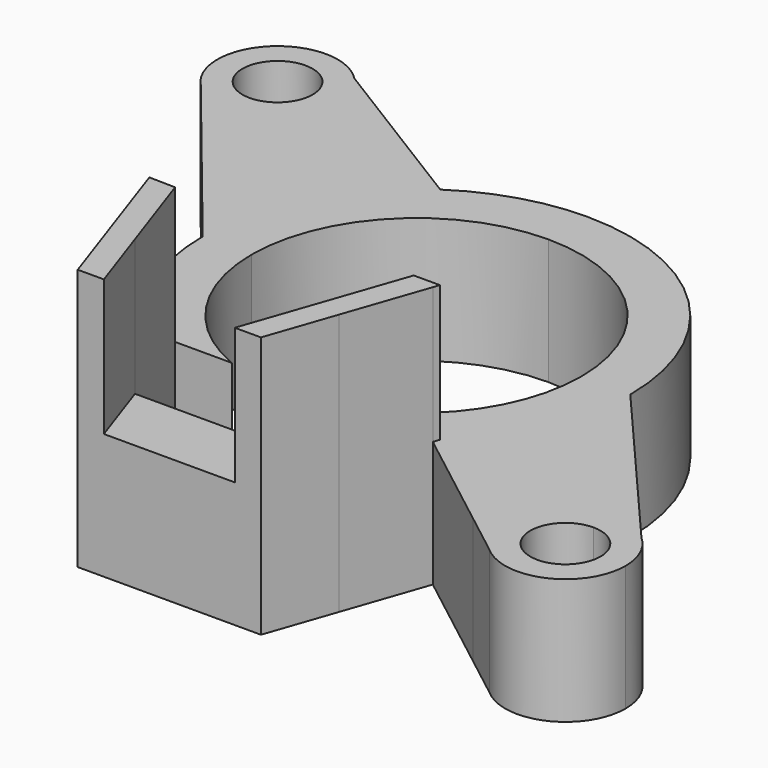
from build123d import *

# Parameters (mm, degrees)
F1_DEPTH = 12
F2_DEPTH = 25
F3_DEPTH = 12


# Not quite as in the source:
# - ends of sketch curves that miss each other by under 0.0002 mm in the source are joined


with BuildPart() as f1:
    # F0 (on Top) → F1 (new body)
    with BuildSketch(Plane.XY):
        with BuildLine():
            ThreePointArc((-53.4150354708, 40.5196217052), (-52.7133447942, 39.4447339634), (-52.4674114416, 38.1848648238))
            Line((-52.4674114416, 38.1848648238), (-50.0674114416, 38.1848649627))
            ThreePointArc((-50.0674114416, 38.1848649627), (-50.4895358529, 40.3473267799), (-51.6939302977, 42.1922833515))
            Line((-51.6939302977, 42.1922833515), (-53.4150354708, 40.5196217052))
        make_face()
        with BuildLine():
            Line((-50.0674114416, 38.1848649627), (-52.4674114416, 38.1848649047))
            ThreePointArc((-52.4674114416, 38.1848649047), (-53.4486037246, 35.8160571069), (-55.8174114415, 34.8348648238))
            Line((-55.8174114415, 34.8348648238), (-55.8174114415, 32.4348648238))
            ThreePointArc((-55.8174114415, 32.4348648238), (-51.7515474497, 34.119000832), (-50.0674114416, 38.1848649627))
        make_face()
        with BuildLine():
            ThreePointArc((-51.6939302977, 42.1922833515), (-50.4895358529, 40.3473267799), (-50.0674114416, 38.1848648238))
            Line((-50.0674114416, 38.1848648238), (-45.2079510631, 38.1848650801))
            Line((-45.2079510631, 38.1848650801), (-51.6939302977, 42.1922833515))
        make_face()
        with BuildLine():
            Line((-45.2079510631, 38.1848650801), (-50.0674114416, 38.1848649627))
            ThreePointArc((-50.0674114416, 38.1848649627), (-51.7515474497, 34.119000832), (-55.8174114415, 32.4348648238))
            Line((-55.8174114415, 32.4348648238), (-55.8174114414, 29.083605512))
            Line((-55.8174114414, 29.083605512), (-44.5532578407, 15.1687110318))
            ThreePointArc((-44.5532578407, 15.1687110318), (-42.1350647352, 24.8048651036), (-35.4555304308, 32.1592477879))
            Line((-35.4555304308, 32.1592477879), (-45.2079510631, 38.1848650801))
        make_face()
        with BuildLine():
            Line((-55.8174114415, 32.4348648238), (-55.8174114415, 34.8348648238))
            ThreePointArc((-55.8174114415, 34.8348648238), (-57.1214560051, 35.0990962362), (-58.2197874124, 35.8501079425))
            Line((-58.2197874124, 35.8501079425), (-59.9408925855, 34.1774462962))
            ThreePointArc((-59.9408925855, 34.1774462962), (-58.0556968865, 32.8883963526), (-55.8174114415, 32.4348648238))
        make_face()
        with BuildLine():
            ThreePointArc((-58.2197874124, 35.8501079425), (-58.1521683229, 40.5872407946), (-53.4150354708, 40.5196217052))
            Line((-53.4150354708, 40.5196217052), (-51.6939302977, 42.1922833515))
            ThreePointArc((-51.6939302977, 42.1922833515), (-59.8248299692, 42.3083459677), (-59.9408925855, 34.1774462962))
            Line((-59.9408925855, 34.1774462962), (-58.2197874124, 35.8501079425))
        make_face()
        with BuildLine():
            Line((-55.8174114414, 29.083605512), (-55.8174114415, 32.4348648238))
            ThreePointArc((-55.8174114415, 32.4348648238), (-58.0556968865, 32.8883963526), (-59.9408925855, 34.1774462962))
            Line((-59.9408925855, 34.1774462962), (-55.8174114414, 29.083605512))
        make_face()
        with BuildLine():
            ThreePointArc((-24.1338443596, 35.5853722206), (-30.0482104313, 34.7100811604), (-35.4555304308, 32.1592477879))
            ThreePointArc((-35.4555304308, 32.1592477879), (-42.1350647352, 24.8048651036), (-44.5532578407, 15.1687110318))
            Line((-44.5532578407, 15.1687110318), (-42.6338443592, 15.1659585535))
            Line((-42.6338443592, 15.1659585535), (-39.8838443592, 15.1659585535))
            ThreePointArc((-39.8838443592, 15.1659585535), (-35.270776163, 26.3028903571), (-24.1338443595, 30.9159585535))
            Line((-24.1338443595, 30.9159585535), (-24.1338443596, 35.5853722206))
        make_face()
        with BuildLine():
            ThreePointArc((-3.7144306922, 15.1659585535), (-9.6951384875, 29.6046644255), (-24.1338443596, 35.5853722206))
            Line((-24.1338443596, 35.5853722206), (-24.1338443595, 30.9159585535))
            ThreePointArc((-24.1338443595, 30.9159585535), (-12.9969125556, 26.3028903573), (-8.3838443592, 15.1659585535))
            Line((-8.3838443592, 15.1659585535), (-5.6338443592, 15.1659585535))
            Line((-5.6338443592, 15.1659585535), (-3.7144306922, 15.1659585535))
        make_face()
        with BuildLine():
            Line((-42.6338443592, 15.1659585535), (-44.5532578407, 15.1687110318))
            ThreePointArc((-44.5532578407, 15.1687110318), (-42.7914410163, 6.8685769492), (-37.807970261, 0.0011725238))
            Line((-37.807970261, 0.0011725238), (-38.0284454354, 0.643162408))
            Line((-38.0284454354, 0.643162408), (-35.5289696075, 0.5919707473))
            Line((-35.5289696075, 0.5919707473), (-42.6338443592, 15.1659585535))
        make_face()
        with BuildLine():
            Line((7.5497227229, 2.079326472), (-3.7144306922, 15.1659585535))
            Line((-3.7144306922, 15.1659585535), (-5.6338443592, 15.1659585535))
            Line((-5.6338443592, 15.1659585535), (-12.7387191109, 0.5919707473))
            Line((-12.7387191109, 0.5919707473), (-10.2387191109, 0.5919707473))
            Line((-10.2387191109, 0.5919707473), (-10.4427343672, 0))
            Line((-10.4427343672, 0), (-0.3331204375, -7.8151351762))
            Line((-0.3331204375, -7.8151351762), (1.9170354556, -7.8151351762))
            ThreePointArc((1.9170354556, -7.8151351762), (3.0939956275, -3.0251503303), (7.549722723, -0.909568585))
            Line((7.549722723, -0.909568585), (7.5497227229, 2.079326472))
        make_face()
        with BuildLine():
            Line((-39.8838443592, 15.1659585535), (-42.6338443592, 15.1659585535))
            Line((-42.6338443592, 15.1659585535), (-35.5289696075, 0.5919707473))
            Line((-35.5289696075, 0.5919707473), (-30.1055593076, 0.5919707473))
            ThreePointArc((-30.1055593076, 0.5919707473), (-37.2127780015, 6.3907665453), (-39.8838443592, 15.1659585535))
        make_face()
        Polygon((-38.0284454354, 0.643162408), (-37.807970261, 0.0011725238), (-35.1236572441, -7.8151351762), (-32.6315665225, -7.8151351762), (-35.5289696075, 0.5919707473), align=None)
        with BuildLine():
            Line((-5.6338443592, 15.1659585535), (-8.3838443592, 15.1659585535))
            ThreePointArc((-8.3838443592, 15.1659585535), (-11.054910717, 6.3907665453), (-18.1621294109, 0.5919707473))
            Line((-18.1621294109, 0.5919707473), (-12.7387191109, 0.5919707473))
            Line((-12.7387191109, 0.5919707473), (-5.6338443592, 15.1659585535))
        make_face()
        with BuildLine():
            Line((11.3813838275, -2.3722765282), (7.5497227229, 2.079326472))
            Line((7.5497227229, 2.079326472), (7.549722723, -0.909568585))
            ThreePointArc((7.549722723, -0.909568585), (9.6004019609, -1.2876774223), (11.3813838275, -2.3722765282))
        make_face()
        Polygon((-32.6315665225, -7.8151351762), (-35.1236572441, -7.8151351762), (-32.8838443592, -14.3371266833), (-30.3838443592, -14.3371266833), align=None)
        Polygon((-10.2387191109, 0.5919707473), (-12.7387191109, 0.5919707473), (-15.636122196, -7.8151351762), (-13.136122196, -7.8151351762), (-10.4427343672, 0), align=None)
        with BuildLine():
            ThreePointArc((11.3813838275, -2.3722765282), (9.6004019609, -1.2876774223), (7.549722723, -0.909568585))
            Line((7.549722723, -0.909568585), (7.549722723, -3.309568585))
            ThreePointArc((7.549722723, -3.309568585), (8.744466279, -3.5298580815), (9.7820818013, -4.1617549519))
            Line((9.7820818013, -4.1617549519), (11.3813838275, -2.3722765282))
        make_face()
        with BuildLine():
            Line((7.549722723, -3.309568585), (7.549722723, -0.909568585))
            ThreePointArc((7.549722723, -0.909568585), (3.0939956275, -3.0251503303), (1.9170354556, -7.8151351762))
            ThreePointArc((1.9170354556, -7.8151351762), (2.5652068364, -9.5261172721), (3.7180616186, -10.9468606418))
            Line((3.7180616186, -10.9468606418), (5.3173636448, -9.1573822181))
            ThreePointArc((5.3173636448, -9.1573822181), (4.4200122196, -5.464825029), (7.549722723, -3.309568585))
        make_face()
        with BuildLine():
            ThreePointArc((13.2997227231, -6.659568585), (12.7982725871, -4.3111171112), (11.3813838275, -2.3722765282))
            Line((11.3813838275, -2.3722765282), (9.7820818013, -4.1617549519))
            ThreePointArc((9.7820818013, -4.1617549519), (10.6075735134, -5.2913403351), (10.8997227231, -6.659568585))
            ThreePointArc((10.8997227231, -6.659568585), (8.917950973, -9.7174193754), (5.3173636448, -9.1573822181))
            Line((5.3173636448, -9.1573822181), (3.7180616186, -10.9468606418))
            ThreePointArc((3.7180616186, -10.9468606418), (9.8981741968, -11.908118449), (13.2997227231, -6.659568585))
        make_face()
        Polygon((-24.1338443592, -7.8151351762), (-32.6315665225, -7.8151351762), (-30.3838443592, -14.3371266833), (-24.1338443592, -14.3371266833), (-24.1338443592, -7.8529477167), align=None)
        Polygon((-13.136122196, -7.8151351762), (-15.636122196, -7.8151351762), (-17.8838443592, -14.3371266833), (-15.3838443592, -14.3371266833), align=None)
        Polygon((-17.8838443592, -14.3371266833), (-15.636122196, -7.8151351762), (-24.1338443592, -7.8151351762), (-24.1338443592, -7.8529477167), (-24.1338443592, -14.3371266833), align=None)
    extrude(amount=F1_DEPTH)

    # F0 (on Top) → F2 (join)
    with BuildSketch(Plane.XY):
        Polygon((-38.0284454354, 0.643162408), (-37.807970261, 0.0011725238), (-35.1236572441, -7.8151351762), (-32.6315665225, -7.8151351762), (-35.5289696075, 0.5919707473), align=None)
        Polygon((-32.6315665225, -7.8151351762), (-35.1236572441, -7.8151351762), (-32.8838443592, -14.3371266833), (-30.3838443592, -14.3371266833), align=None)
        Polygon((-13.136122196, -7.8151351762), (-15.636122196, -7.8151351762), (-17.8838443592, -14.3371266833), (-15.3838443592, -14.3371266833), align=None)
        Polygon((-10.2387191109, 0.5919707473), (-12.7387191109, 0.5919707473), (-15.636122196, -7.8151351762), (-13.136122196, -7.8151351762), (-10.4427343672, 0), align=None)
    extrude(amount=F2_DEPTH)

    # F0 (on Top) → F3 (join)
    with BuildSketch(Plane.XY):
        with BuildLine():
            ThreePointArc((3.7180616186, -10.9468606418), (2.5652068364, -9.5261172721), (1.9170354556, -7.8151351762))
            Line((1.9170354556, -7.8151351762), (-0.3331204375, -7.8151351762))
            Line((-0.3331204375, -7.8151351762), (3.7180616186, -10.9468606418))
        make_face()
    extrude(amount=F3_DEPTH)


solid = f1.part
